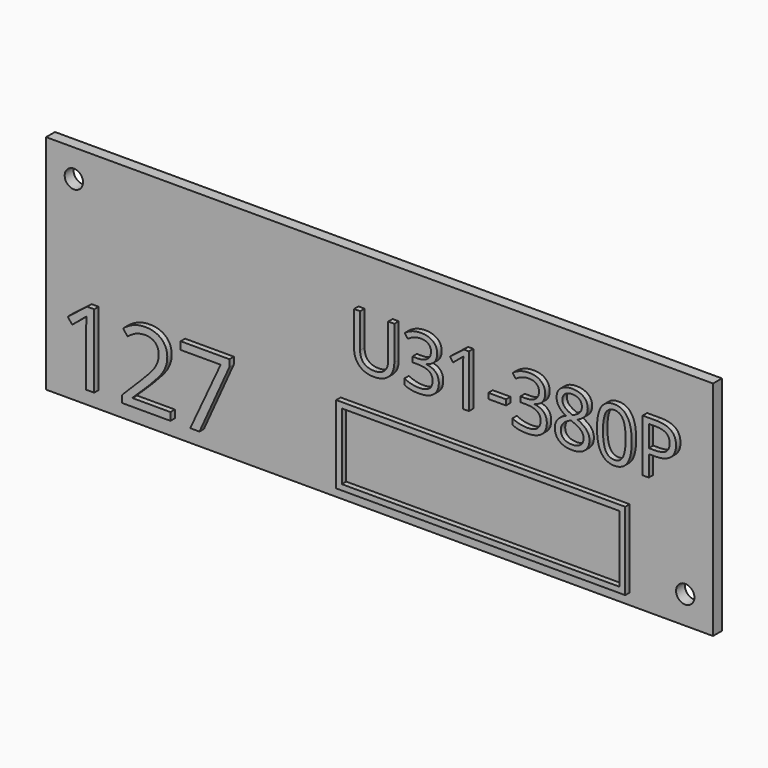
from build123d import *

# Parameters (mm, degrees)
F0_W         = 120
F0_H         = 40
F1_DEPTH     = 2
F3_D         = 3.3
F4_TEXT_SIZE = 13.2628743135
F5_DEPTH     = 1
F6_TEXT_SIZE = 18.5054667028
F7_DEPTH     = 1
F8_W         = 52
F8_H         = 14
F8_W_2       = 49.99999962
F8_H_2       = 11.99999962
F9_DEPTH     = 1


# Not quite as in the source:
# - Text() gives the source's letters only with a copy of the font that has no kerning and outlines rounded to 1/6400 em; it was checked with that copy


with BuildPart() as f1:
    # F0 (on Front) → F1 (new body)
    with BuildSketch(Plane.XZ):
        Rectangle(F0_W, F0_H)
    extrude(amount=F1_DEPTH)

    # F3 (through all)
    with Locations(Plane.XZ.offset(2)):
        with Locations((-55, 15), (55, -15)):
            Hole(F3_D / 2)

    # F4 (on face) → F5 (join)
    with BuildSketch(Plane.XZ.offset(2)):
        with Locations((-5, 2)):
            Text('U31-380P', F4_TEXT_SIZE, font='Open Sans', text_align=(TextAlign.LEFT, TextAlign.BOTTOM))
    extrude(amount=F5_DEPTH)

    # F6 (on face) → F7 (join)
    with BuildSketch(Plane.XZ.offset(2)):
        with Locations((-57, -17)):
            Text('127', F6_TEXT_SIZE, font='Open Sans', text_align=(TextAlign.LEFT, TextAlign.BOTTOM))
    extrude(amount=F7_DEPTH)

    # F8 (on face) → F9 (join)
    with BuildSketch(Plane.XZ.offset(2)):
        with Locations((19, -11)):
            Rectangle(F8_W, F8_H)
        with Locations((19, -11)):
            Rectangle(F8_W_2, F8_H_2, mode=Mode.SUBTRACT)
    extrude(amount=F9_DEPTH)


solid = f1.part
